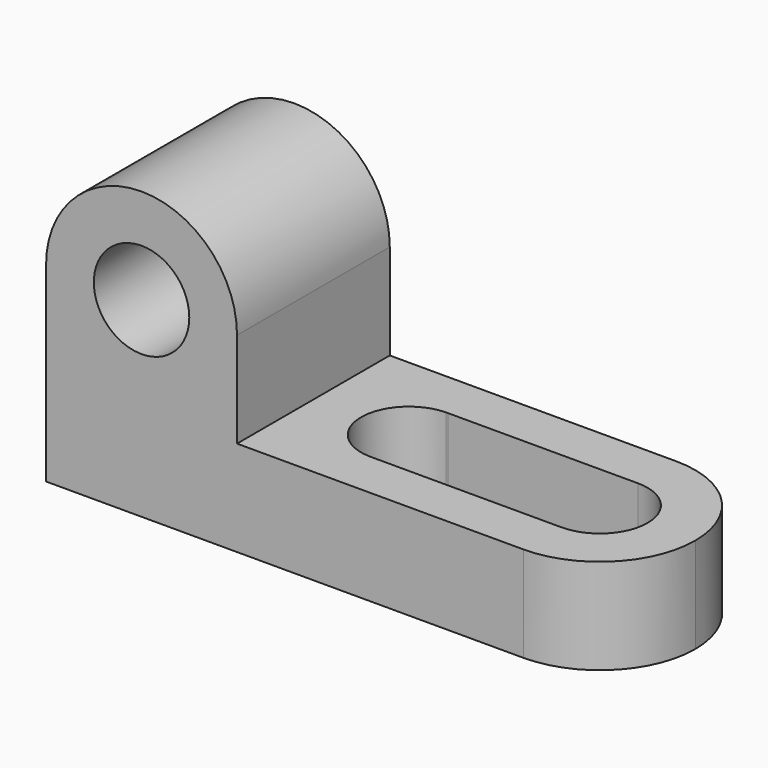
from build123d import *

# Parameters (mm, degrees)
F0_R     = 6.35
F2_DEPTH = 25.4
F3_W     = 25.4
F3_H     = 12.7
F4_DEPTH = 50.8
F5_R     = 12.69999
F7_DEPTH = 25.4


# Not quite as in the source:
# - a fillet or chamfer is up to 0.001 mm smaller than in the source, because OpenCascade refuses the exact size


with BuildPart() as f2:
    # F0 (on Front) → F2 (new body)
    with BuildSketch(Plane.XZ):
        with BuildLine():
            Line((0, 25.4), (0, 0))
            Line((0, 0), (25.4, 0))
            Line((25.4, 0), (25.4, 25.4))
            ThreePointArc((25.4, 25.4), (12.7, 38.1), (0, 25.4))
        make_face()
        with Locations((12.7, 25.4)):
            Circle(F0_R, mode=Mode.SUBTRACT)
    extrude(amount=-F2_DEPTH)

    # F3 (on face) → F4 (join)
    with BuildSketch(Plane.YZ.offset(25.4)):
        with Locations((12.7, 6.35)):
            Rectangle(F3_W, F3_H)
    extrude(amount=F4_DEPTH)

    # F5 (radius 12.7 in the source; OpenCascade refuses exactly that, so slightly less here)
    f5_edges = [f2.edges().sort_by_distance(p)[0] for p in [
        (76.2, 0, 6.35),
        (76.2, 25.4, 6.35),
    ]]
    fillet(f5_edges, radius=F5_R)

    # F6 (on face) → F7 (cut)
    with BuildSketch(Plane.XY.offset(12.7)):
        with BuildLine():
            Line((38.2369286846, 19.0485234925), (37.9623292283, 19.0485074434))
            ThreePointArc((37.9623292283, 19.0485074434), (31.7500032955, 12.7064693713), (37.9493938195, 6.3517862529))
            Line((37.9493938195, 6.3517862529), (38.2497185591, 6.3517652569))
            ThreePointArc((38.2497185591, 6.3517652569), (42.6427531768, 8.26312119), (44.45, 12.7))
            ThreePointArc((44.45, 12.7), (42.638281456, 17.1414526257), (38.2369286846, 19.0485234925))
        make_face()
        with BuildLine():
            Line((63.4996288697, 19.0499999892), (38.2369286846, 19.0485234925))
            ThreePointArc((38.2369286846, 19.0485234925), (42.638281456, 17.1414526257), (44.45, 12.7))
            ThreePointArc((44.45, 12.7), (42.6427531768, 8.26312119), (38.2497185591, 6.3517652569))
            Line((38.2497185591, 6.3517652569), (63.4995560651, 6.3500000155))
            ThreePointArc((63.4995560651, 6.3500000155), (57.1500000001, 12.7000364023), (63.4996288697, 19.0499999892))
        make_face()
        with BuildLine():
            ThreePointArc((69.85, 12.7), (67.9899968442, 17.190259273), (63.4996288697, 19.0499999892))
            ThreePointArc((63.4996288697, 19.0499999892), (57.1500000001, 12.7000364023), (63.4995560651, 6.3500000155))
            ThreePointArc((63.4995560651, 6.3500000155), (67.9899711031, 8.2097149875), (69.85, 12.7))
        make_face()
    extrude(amount=-F7_DEPTH, mode=Mode.SUBTRACT)


solid = f2.part
